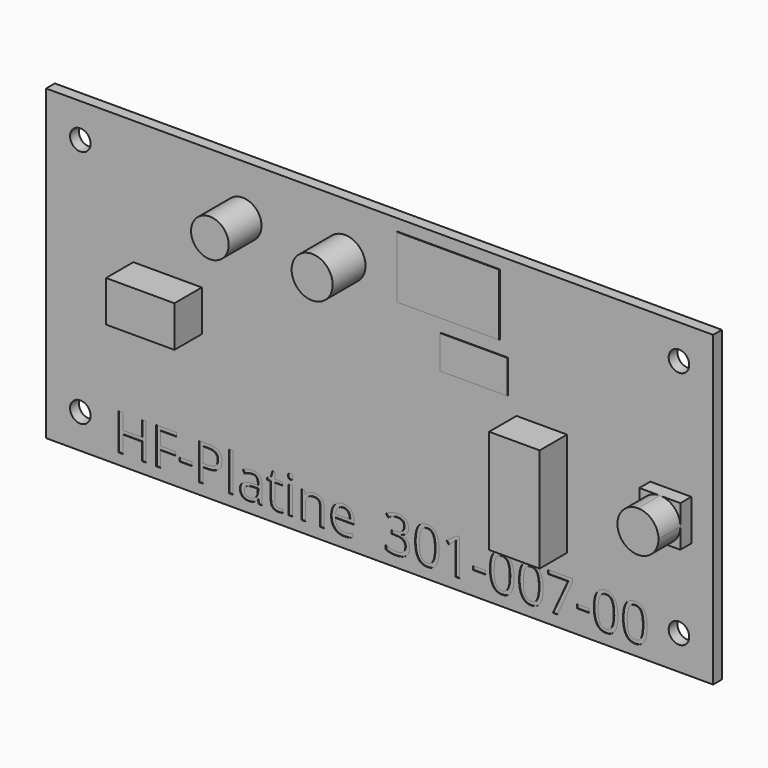
from build123d import *

# Parameters (mm, degrees)
F0_W         = 97.5
F0_H         = 45
F0_R         = 1.5
F0_W_2       = 7.3819365352
F0_H_2       = 15.2102245484
F0_W_3       = 10
F0_H_3       = 6
F0_R_2       = 2.75
F0_R_3       = 3
F0_W_4       = 9.8289120942
F0_H_4       = 4.8918086104
F0_W_5       = 14.9580829311
F0_H_5       = 9.0310713276
F1_DEPTH     = 1.6
F2_TEXT_SIZE = 7.4598705396
F3_DEPTH     = 0.1
F4_DEPTH     = 0.1
F5_DEPTH     = 5
F6_DEPTH     = 2
F7_DEPTH     = 6
F8_DEPTH     = 6


# Not quite as in the source:
# - a feature names something its author has since deleted; it is built from what else it names
# - Text() gives the source's letters only with a copy of the font that has no kerning and outlines rounded to 1/6400 em; it was checked with that copy


with BuildPart() as f1:
    # F0 (on Front) → F1 (new body)
    with BuildSketch(Plane.XZ):
        Rectangle(F0_W, F0_H)
        with Locations((-43.75, -17.5)):
            Circle(F0_R, mode=Mode.SUBTRACT)
        with Locations((43.75, -17.5)):
            Circle(F0_R, mode=Mode.SUBTRACT)
        with Locations((23.7008733675, -4.8805511324)):
            Rectangle(F0_W_2, F0_H_2, mode=Mode.SUBTRACT)
        Polygon((45.5568409264, 0.625289252), (45.5568409264, -2.374710748), (45.5568409264, -5.374710748), (42.5568409264, -5.374710748), (39.5568409264, -5.374710748), (39.5568409264, -2.374710748), (39.5568409264, 0.625289252), (42.5568409264, 0.625289252), align=None, mode=Mode.SUBTRACT)
        with Locations((-30.9898284078, 1.2968331836)):
            Rectangle(F0_W_3, F0_H_3, mode=Mode.SUBTRACT)
        with Locations((-43.75, 17.5)):
            Circle(F0_R, mode=Mode.SUBTRACT)
        with Locations((-20.0124884674, 15.0544113171)):
            Circle(F0_R_2, mode=Mode.SUBTRACT)
        with Locations((-5.0621527245, 14.864595566)):
            Circle(F0_R_3, mode=Mode.SUBTRACT)
        with Locations((13.8343656436, 7.3748065624)):
            Rectangle(F0_W_4, F0_H_4, mode=Mode.SUBTRACT)
        with Locations((10.0832929602, 16.2711669691)):
            Rectangle(F0_W_5, F0_H_5, mode=Mode.SUBTRACT)
        with Locations((43.75, 17.5)):
            Circle(F0_R, mode=Mode.SUBTRACT)
        with Locations((-30.9898284078, 1.2968331836)):
            Rectangle(F0_W_3, F0_H_3)
        with Locations((23.7008733675, -4.8805511324)):
            Rectangle(F0_W_2, F0_H_2)
        with Locations((10.0832929602, 16.2711669691)):
            Rectangle(F0_W_5, F0_H_5)
        with Locations((-5.0621527245, 14.864595566)):
            Circle(F0_R_3)
        with Locations((-20.0124884674, 15.0544113171)):
            Circle(F0_R_2)
        with BuildLine():
            ThreePointArc((42.5568409264, -5.374710748), (44.67816127, -4.4960310915), (45.5568409264, -2.374710748))
            ThreePointArc((45.5568409264, -2.374710748), (44.67816127, -0.2533904044), (42.5568409264, 0.625289252))
            ThreePointArc((42.5568409264, 0.625289252), (40.4355205828, -0.2533904044), (39.5568409264, -2.374710748))
            ThreePointArc((39.5568409264, -2.374710748), (40.4355205828, -4.4960310915), (42.5568409264, -5.374710748))
        make_face()
        with BuildLine():
            Line((45.5568409264, -5.374710748), (45.5568409264, -2.374710748))
            ThreePointArc((45.5568409264, -2.374710748), (44.67816127, -4.4960310915), (42.5568409264, -5.374710748))
            Line((42.5568409264, -5.374710748), (45.5568409264, -5.374710748))
        make_face()
        with BuildLine():
            ThreePointArc((42.5568409264, 0.625289252), (44.67816127, -0.2533904044), (45.5568409264, -2.374710748))
            Line((45.5568409264, -2.374710748), (45.5568409264, 0.625289252))
            Line((45.5568409264, 0.625289252), (42.5568409264, 0.625289252))
        make_face()
        with BuildLine():
            ThreePointArc((39.5568409264, -2.374710748), (40.4355205828, -0.2533904044), (42.5568409264, 0.625289252))
            Line((42.5568409264, 0.625289252), (39.5568409264, 0.625289252))
            Line((39.5568409264, 0.625289252), (39.5568409264, -2.374710748))
        make_face()
        with BuildLine():
            Line((39.5568409264, -5.374710748), (42.5568409264, -5.374710748))
            ThreePointArc((42.5568409264, -5.374710748), (40.4355205828, -4.4960310915), (39.5568409264, -2.374710748))
            Line((39.5568409264, -2.374710748), (39.5568409264, -5.374710748))
        make_face()
        with Locations((13.8343656436, 7.3748065624)):
            Rectangle(F0_W_4, F0_H_4)
    extrude(amount=-F1_DEPTH)

    # F2 (on face) → F3 (cut)
    with BuildSketch(Plane.XZ):
        with Locations((-38.8893261552, -20.8913153037)):
            Text('HF-Platine  301-007-00', F2_TEXT_SIZE, font='Open Sans', text_align=(TextAlign.LEFT, TextAlign.BOTTOM))
    extrude(amount=-F3_DEPTH, mode=Mode.SUBTRACT)

    # F0 (on Front) → F4 (join)
    with BuildSketch(Plane.XZ):
        with Locations((10.0832929602, 16.2711669691)):
            Rectangle(F0_W_5, F0_H_5)
        with Locations((13.8343656436, 7.3748065624)):
            Rectangle(F0_W_4, F0_H_4)
    extrude(amount=F4_DEPTH)

    # F0 (on Front) → F5 (join)
    with BuildSketch(Plane.XZ):
        with Locations((-30.9898284078, 1.2968331836)):
            Rectangle(F0_W_3, F0_H_3)
        with Locations((23.7008733675, -4.8805511324)):
            Rectangle(F0_W_2, F0_H_2)
    extrude(amount=F5_DEPTH)

    # F0 (on Front) → F8 (join)
    with BuildSketch(Plane.XZ):
        with Locations((-20.0124884674, 15.0544113171)):
            Circle(F0_R_2)
        with Locations((-5.0621527245, 14.864595566)):
            Circle(F0_R_3)
    extrude(amount=F8_DEPTH)


with BuildPart() as f6:
    # F0 (on Front) → F6 (new body)
    with BuildSketch(Plane.XZ):
        with BuildLine():
            Line((39.5568409264, -5.374710748), (42.5568409264, -5.374710748))
            ThreePointArc((42.5568409264, -5.374710748), (40.4355205828, -4.4960310915), (39.5568409264, -2.374710748))
            Line((39.5568409264, -2.374710748), (39.5568409264, -5.374710748))
        make_face()
        with BuildLine():
            ThreePointArc((39.5568409264, -2.374710748), (40.4355205828, -0.2533904044), (42.5568409264, 0.625289252))
            Line((42.5568409264, 0.625289252), (39.5568409264, 0.625289252))
            Line((39.5568409264, 0.625289252), (39.5568409264, -2.374710748))
        make_face()
        with BuildLine():
            ThreePointArc((42.5568409264, 0.625289252), (44.67816127, -0.2533904044), (45.5568409264, -2.374710748))
            Line((45.5568409264, -2.374710748), (45.5568409264, 0.625289252))
            Line((45.5568409264, 0.625289252), (42.5568409264, 0.625289252))
        make_face()
        with BuildLine():
            Line((45.5568409264, -5.374710748), (45.5568409264, -2.374710748))
            ThreePointArc((45.5568409264, -2.374710748), (44.67816127, -4.4960310915), (42.5568409264, -5.374710748))
            Line((42.5568409264, -5.374710748), (45.5568409264, -5.374710748))
        make_face()
        with BuildLine():
            ThreePointArc((42.5568409264, -5.374710748), (44.67816127, -4.4960310915), (45.5568409264, -2.374710748))
            ThreePointArc((45.5568409264, -2.374710748), (44.67816127, -0.2533904044), (42.5568409264, 0.625289252))
            ThreePointArc((42.5568409264, 0.625289252), (40.4355205828, -0.2533904044), (39.5568409264, -2.374710748))
            ThreePointArc((39.5568409264, -2.374710748), (40.4355205828, -4.4960310915), (42.5568409264, -5.374710748))
        make_face()
    extrude(amount=F6_DEPTH)

    # F0 (on Front) → F7 (join)
    with BuildSketch(Plane.XZ):
        with BuildLine():
            ThreePointArc((42.5568409264, -5.374710748), (44.67816127, -4.4960310915), (45.5568409264, -2.374710748))
            ThreePointArc((45.5568409264, -2.374710748), (44.67816127, -0.2533904044), (42.5568409264, 0.625289252))
            ThreePointArc((42.5568409264, 0.625289252), (40.4355205828, -0.2533904044), (39.5568409264, -2.374710748))
            ThreePointArc((39.5568409264, -2.374710748), (40.4355205828, -4.4960310915), (42.5568409264, -5.374710748))
        make_face()
    extrude(amount=F7_DEPTH)


solid = Compound([f1.part, f6.part])
